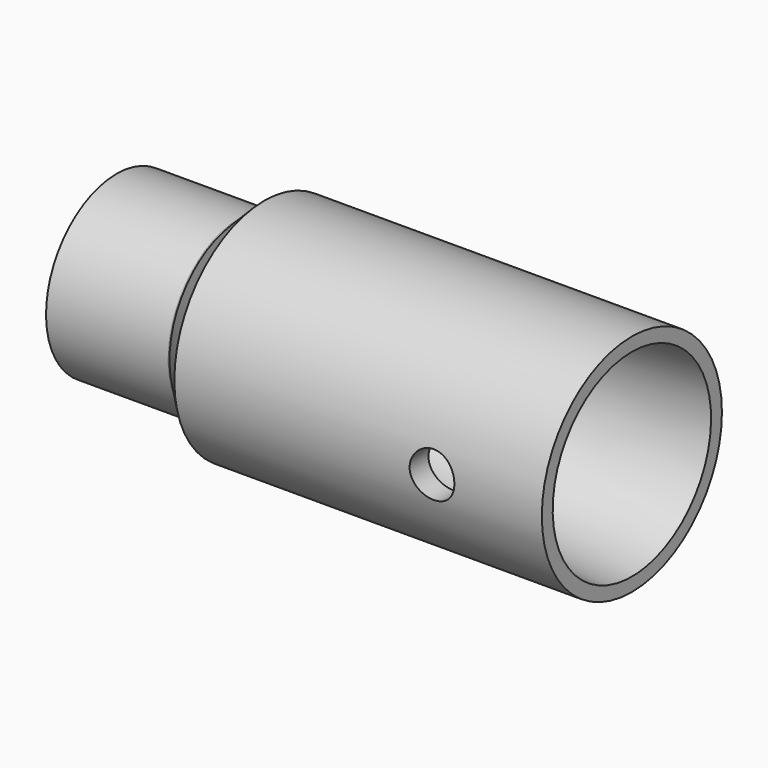
from build123d import *

# Parameters (mm, degrees)
F2_S5_R     = 6.5
F2_T6_DEPTH = 13
F4_DEPTH    = 10
F5_R        = 1.65
F6_DEPTH    = 8.301


# Not quite as in the source:
# - a fillet or chamfer that OpenCascade refuses, or shapes differently, is made with other operations: its cross-section is extruded or revolved along the edge and cut away or added


with BuildPart() as f1:
    # F0 (on Front) → F1 (revolve)
    with BuildSketch(Plane.XZ):
        Polygon((0, 6.5), (0, 4.95), (9.6, 4.95), (10, 4.55), (11, 4.55), (11, 5.25), (38, 7.3), (38, 8.3), (9, 8.3), (9, 6.5), align=None)
    revolve(axis=Axis((19, 0, 0), (1, 0, 0)))

    # F2: chamfer of 1.9 on 1 edges, made by hand


with BuildPart() as f2_tool2:
    # F2_s3 → F2_t4 (revolve)
    with BuildSketch(Plane.XZ):
        Polygon((10.9, 8.3), (9, 6.4), (9, 8.3), align=None)
    revolve(axis=Axis((9, 0, 0), (1, 0, 0)))

    # F2_s5 → F2_t6 (cut, symmetric)
    with BuildSketch(Plane.YZ.offset(9.9)):
        Circle(F2_S5_R)
    extrude(amount=F2_T6_DEPTH, both=True, mode=Mode.SUBTRACT)


with BuildPart() as f1_1:
    add(f1.part)

    # F2_t1: cut F2_tool2
    add(f2_tool2.part, mode=Mode.SUBTRACT)

    # F3 (on face) → F4 (cut)
    with BuildSketch(Plane.YZ.offset(11)):
        with BuildLine():
            Line((-4.6153846154, 2.502144051), (-4, 2.1685248442))
            ThreePointArc((-4, 2.1685248442), (0, 4.55), (4, 2.1685248442))
            Line((4, 2.1685248442), (4.6153846154, 2.502144051))
            ThreePointArc((4.6153846154, 2.502144051), (0, 5.25), (-4.6153846154, 2.502144051))
        make_face()
    extrude(amount=-F4_DEPTH, mode=Mode.SUBTRACT)

    # F5 (on Front) → F6 (cut, through all)
    with BuildSketch(Plane.XZ):
        with Locations((29.9, 0)):
            Circle(F5_R)
    extrude(amount=F6_DEPTH, mode=Mode.SUBTRACT)


solid = f1_1.part
